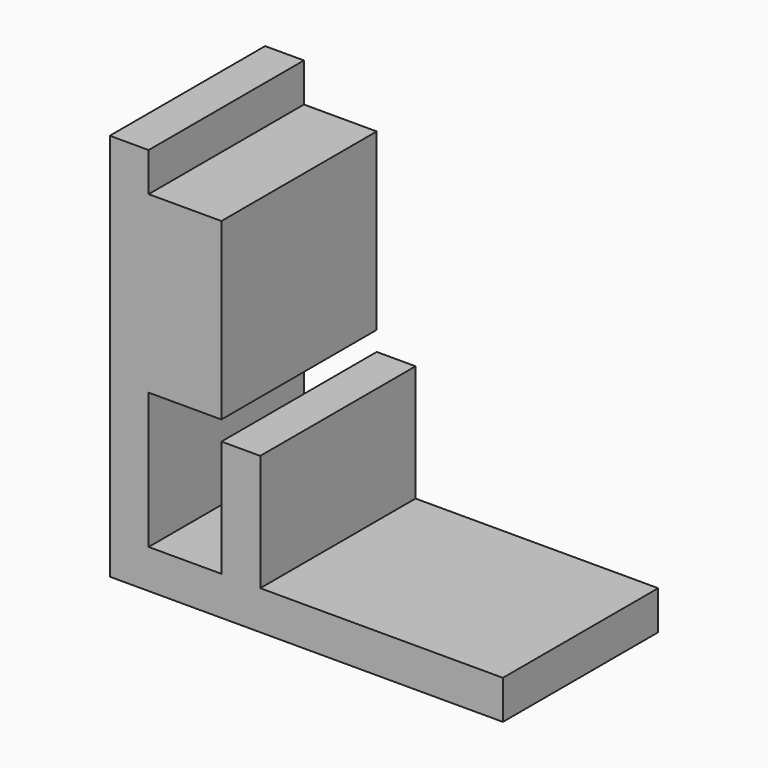
from build123d import *

# Parameters (mm, degrees)
F1_DEPTH = 40


# Not quite as in the source:
# - a feature names something its author has since deleted; it is built from what else it names


with BuildPart() as f1:
    # F0 (on Front) → F1 (new body)
    with BuildSketch(Plane.XZ):
        Polygon((23, 72), (8, 72), (8, 39.8151502013), (8, 36), (23, 36), align=None)
        Polygon((0, 80), (0, 0), (81, 0), (81, 8), (56, 8), (31, 8), (31, 32), (23, 32), (23, 8), (8, 8), (8, 36), (8, 39.8151502013), (8, 72), (8, 80), align=None)
    extrude(amount=-F1_DEPTH)


solid = f1.part
